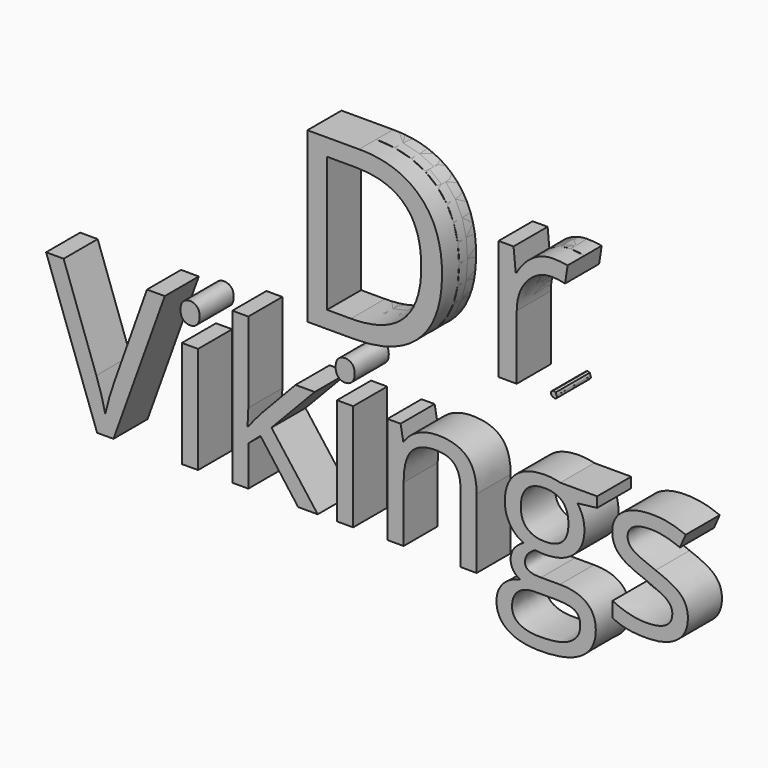
from build123d import *

# Parameters (mm, degrees)
F0_TEXT_SIZE   = 140.9615354431
F0_TEXT_SIZE_2 = 133.6603735884
F1_DEPTH       = 12.7
F2_TEXT_SIZE   = 118.9749894871
F3_DEPTH       = 25.4
F4_DEPTH       = 25.4


# Not quite as in the source:
# - Text() gives the source's letters only with a copy of the font that has no kerning and outlines rounded to 1/6400 em; it was checked with that copy


with BuildPart() as f1:
    # F0 (on Front) → F1 (new body)
    with BuildSketch(Plane.XZ):
        with BuildLine():
            Line((42.0875150615, 1.5779257073), (42.1086192093, 1.6124475888))
            Line((42.1086192093, 1.6124475888), (41.5891754677, 3.0403819103))
            Line((41.5891754677, 3.0403819103), (40.1489035847, 3.5245669269))
            Line((40.1489035847, 3.5245669269), (38.8723576644, 2.7004014456))
            Line((38.8723576644, 2.7004014456), (38.7208028216, 1.1884988836))
            Line((38.7208028216, 1.1884988836), (39.808362944, 0.1273527073))
            Line((39.808362944, 0.1273527073), (40.3411542105, 0.1940257916))
            add(Edge.make_bspline(
                [(40.3411542105, 0.1940257916), (40.1928909038, 0.4557004277), (40.1928909038, 0.8968516983)],
                knots=[0.2763769785, 0.2763769785, 0.2763769785, 1, 1, 1], degree=2))
            add(Edge.make_bspline(
                [(40.1928909038, 0.8968516983), (40.1928909038, 1.4658512652), (40.4516502307, 1.757124853)],
                knots=[0, 0, 0, 1, 1, 1], degree=2))
            add(Edge.make_bspline(
                [(40.4516502307, 1.757124853), (40.7104095575, 2.0483984408), (41.1927044285, 2.0483984408)],
                knots=[0, 0, 0, 1, 1, 1], degree=2))
            add(Edge.make_bspline(
                [(41.1927044285, 2.0483984408), (41.6831278647, 2.0483984408), (41.9581443221, 1.757124853)],
                knots=[0, 0, 0, 1, 1, 1], degree=2))
            add(Edge.make_bspline(
                [(41.9581443221, 1.757124853), (42.0330234032, 1.6778194222), (42.0875150615, 1.5779257073)],
                knots=[0, 0, 0, 0.2722712738, 0.2722712738, 0.2722712738], degree=2))
        make_face()
        with BuildLine():
            add(Edge.make_bspline(
                [(42.0875150615, 1.5779257073), (42.2331607794, 1.3109290283), (42.2331607794, 0.8968516983)],
                knots=[0.2722712738, 0.2722712738, 0.2722712738, 1, 1, 1], degree=2))
            Line((42.0875150615, 1.5779257073), (41.3160830774, 0.316027631))
            Line((41.3160830774, 0.316027631), (40.3411542105, 0.1940257916))
            add(Edge.make_bspline(
                [(40.4760359264, 0.0203214131), (40.3977811606, 0.0940830823), (40.3411542105, 0.1940257916)],
                knots=[0, 0, 0, 0.2763769785, 0.2763769785, 0.2763769785], degree=2))
            add(Edge.make_bspline(
                [(41.1927044285, -0.246566479), (40.759180949, -0.246566479), (40.4760359264, 0.0203214131)],
                knots=[0, 0, 0, 1, 1, 1], degree=2))
            add(Edge.make_bspline(
                [(41.9540800394, 0.0501261523), (41.6749992995, -0.246566479), (41.1927044285, -0.246566479)],
                knots=[0, 0, 0, 1, 1, 1], degree=2))
            add(Edge.make_bspline(
                [(42.2331607794, 0.8968516983), (42.2331607794, 0.3468187836), (41.9540800394, 0.0501261523)],
                knots=[0, 0, 0, 1, 1, 1], degree=2))
        make_face()
        with BuildLine():
            Line((41.3160830774, 0.316027631), (42.0875150615, 1.5779257073))
            add(Edge.make_bspline(
                [(41.9581443221, 1.757124853), (42.0330234032, 1.6778194222), (42.0875150615, 1.5779257073)],
                knots=[0, 0, 0, 0.2722712738, 0.2722712738, 0.2722712738], degree=2))
            add(Edge.make_bspline(
                [(41.1927044285, 2.0483984408), (41.6831278647, 2.0483984408), (41.9581443221, 1.757124853)],
                knots=[0, 0, 0, 1, 1, 1], degree=2))
            add(Edge.make_bspline(
                [(40.4516502307, 1.757124853), (40.7104095575, 2.0483984408), (41.1927044285, 2.0483984408)],
                knots=[0, 0, 0, 1, 1, 1], degree=2))
            add(Edge.make_bspline(
                [(40.1928909038, 0.8968516983), (40.1928909038, 1.4658512652), (40.4516502307, 1.757124853)],
                knots=[0, 0, 0, 1, 1, 1], degree=2))
            add(Edge.make_bspline(
                [(40.3411542105, 0.1940257916), (40.1928909038, 0.4557004277), (40.1928909038, 0.8968516983)],
                knots=[0.2763769785, 0.2763769785, 0.2763769785, 1, 1, 1], degree=2))
            Line((40.3411542105, 0.1940257916), (41.3160830774, 0.316027631))
        make_face()
        with Locations((-120.3903444111, -8.0557282781)):
            Text('D', F0_TEXT_SIZE, font='Open Sans', text_align=(TextAlign.LEFT, TextAlign.BOTTOM))
        with Locations((-3.9876404893, 0)):
            Text('r', F0_TEXT_SIZE_2, font='Open Sans', text_align=(TextAlign.LEFT, TextAlign.BOTTOM))
    extrude(amount=F1_DEPTH)


with BuildPart() as f3:
    # F2 (on Front) → F3 (new body)
    with BuildSketch(Plane.XZ):
        with Locations((-262.4848634005, -107.1744132787)):
            Text('Vikings', F2_TEXT_SIZE, font='Open Sans', text_align=(TextAlign.LEFT, TextAlign.BOTTOM))
    extrude(amount=F3_DEPTH)


with BuildPart() as f4:
    # F0 (on Front) → F4 (new body)
    with BuildSketch(Plane.XZ):
        with BuildLine():
            Line((42.0875150615, 1.5779257073), (42.1086192093, 1.6124475888))
            Line((42.1086192093, 1.6124475888), (41.5891754677, 3.0403819103))
            Line((41.5891754677, 3.0403819103), (40.1489035847, 3.5245669269))
            Line((40.1489035847, 3.5245669269), (38.8723576644, 2.7004014456))
            Line((38.8723576644, 2.7004014456), (38.7208028216, 1.1884988836))
            Line((38.7208028216, 1.1884988836), (39.808362944, 0.1273527073))
            Line((39.808362944, 0.1273527073), (40.3411542105, 0.1940257916))
            add(Edge.make_bspline(
                [(40.3411542105, 0.1940257916), (40.1928909038, 0.4557004277), (40.1928909038, 0.8968516983)],
                knots=[0.2763769785, 0.2763769785, 0.2763769785, 1, 1, 1], degree=2))
            add(Edge.make_bspline(
                [(40.1928909038, 0.8968516983), (40.1928909038, 1.4658512652), (40.4516502307, 1.757124853)],
                knots=[0, 0, 0, 1, 1, 1], degree=2))
            add(Edge.make_bspline(
                [(40.4516502307, 1.757124853), (40.7104095575, 2.0483984408), (41.1927044285, 2.0483984408)],
                knots=[0, 0, 0, 1, 1, 1], degree=2))
            add(Edge.make_bspline(
                [(41.1927044285, 2.0483984408), (41.6831278647, 2.0483984408), (41.9581443221, 1.757124853)],
                knots=[0, 0, 0, 1, 1, 1], degree=2))
            add(Edge.make_bspline(
                [(41.9581443221, 1.757124853), (42.0330234032, 1.6778194222), (42.0875150615, 1.5779257073)],
                knots=[0, 0, 0, 0.2722712738, 0.2722712738, 0.2722712738], degree=2))
        make_face()
        with BuildLine():
            add(Edge.make_bspline(
                [(42.0875150615, 1.5779257073), (42.2331607794, 1.3109290283), (42.2331607794, 0.8968516983)],
                knots=[0.2722712738, 0.2722712738, 0.2722712738, 1, 1, 1], degree=2))
            Line((42.0875150615, 1.5779257073), (41.3160830774, 0.316027631))
            Line((41.3160830774, 0.316027631), (40.3411542105, 0.1940257916))
            add(Edge.make_bspline(
                [(40.4760359264, 0.0203214131), (40.3977811606, 0.0940830823), (40.3411542105, 0.1940257916)],
                knots=[0, 0, 0, 0.2763769785, 0.2763769785, 0.2763769785], degree=2))
            add(Edge.make_bspline(
                [(41.1927044285, -0.246566479), (40.759180949, -0.246566479), (40.4760359264, 0.0203214131)],
                knots=[0, 0, 0, 1, 1, 1], degree=2))
            add(Edge.make_bspline(
                [(41.9540800394, 0.0501261523), (41.6749992995, -0.246566479), (41.1927044285, -0.246566479)],
                knots=[0, 0, 0, 1, 1, 1], degree=2))
            add(Edge.make_bspline(
                [(42.2331607794, 0.8968516983), (42.2331607794, 0.3468187836), (41.9540800394, 0.0501261523)],
                knots=[0, 0, 0, 1, 1, 1], degree=2))
        make_face()
        with BuildLine():
            Line((41.3160830774, 0.316027631), (42.0875150615, 1.5779257073))
            add(Edge.make_bspline(
                [(41.9581443221, 1.757124853), (42.0330234032, 1.6778194222), (42.0875150615, 1.5779257073)],
                knots=[0, 0, 0, 0.2722712738, 0.2722712738, 0.2722712738], degree=2))
            add(Edge.make_bspline(
                [(41.1927044285, 2.0483984408), (41.6831278647, 2.0483984408), (41.9581443221, 1.757124853)],
                knots=[0, 0, 0, 1, 1, 1], degree=2))
            add(Edge.make_bspline(
                [(40.4516502307, 1.757124853), (40.7104095575, 2.0483984408), (41.1927044285, 2.0483984408)],
                knots=[0, 0, 0, 1, 1, 1], degree=2))
            add(Edge.make_bspline(
                [(40.1928909038, 0.8968516983), (40.1928909038, 1.4658512652), (40.4516502307, 1.757124853)],
                knots=[0, 0, 0, 1, 1, 1], degree=2))
            add(Edge.make_bspline(
                [(40.3411542105, 0.1940257916), (40.1928909038, 0.4557004277), (40.1928909038, 0.8968516983)],
                knots=[0.2763769785, 0.2763769785, 0.2763769785, 1, 1, 1], degree=2))
            Line((40.3411542105, 0.1940257916), (41.3160830774, 0.316027631))
        make_face()
        with Locations((-120.3903444111, -8.0557282781)):
            Text('D', F0_TEXT_SIZE, font='Open Sans', text_align=(TextAlign.LEFT, TextAlign.BOTTOM))
        with Locations((-3.9876404893, 0)):
            Text('r', F0_TEXT_SIZE_2, font='Open Sans', text_align=(TextAlign.LEFT, TextAlign.BOTTOM))
    extrude(amount=F4_DEPTH)


solid = Compound([f1.part, f3.part, f4.part])
